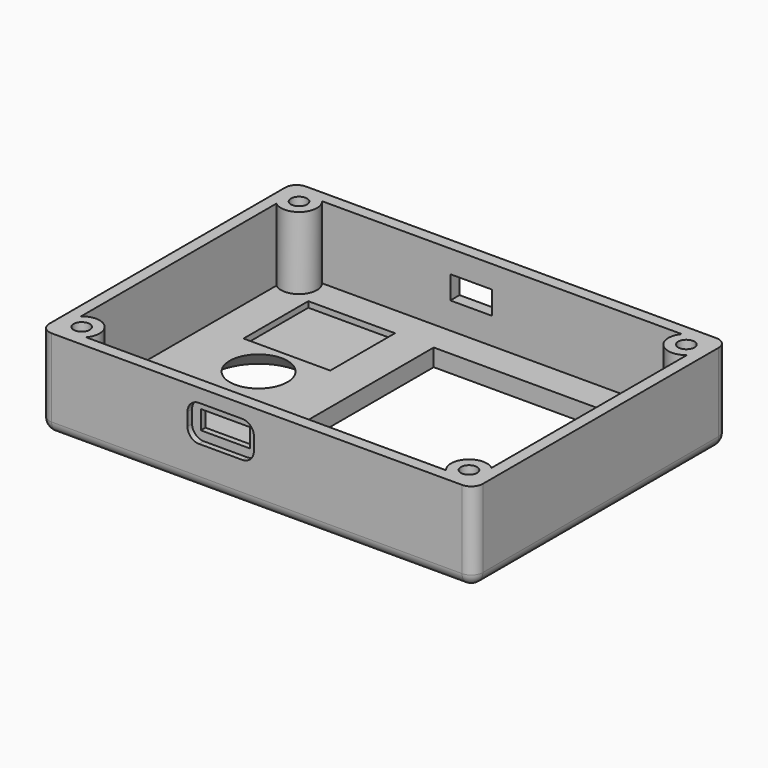
from build123d import *

# Parameters (mm, degrees)
F0_R      = 5
F0_W      = 15
F0_H      = 14
F1_DEPTH  = 3
F0_W_2    = 5
F0_H_2    = 23
F2_DEPTH  = 1
F0_R_2    = 1.4
F3_DEPTH  = 15.5
F4_DEPTH  = 3
F5_R      = 2
F6_W      = 7.25
F6_H      = 4
F7_DEPTH  = 25
F8_W      = 8.5
F8_H      = 3.25
F9_DEPTH  = 25
F8_W_2    = 11.5
F8_H_2    = 6.25
F10_DEPTH = 1
F11_R     = 2
F12_DEPTH = 2
F13_SIZE  = 2.99999


# Not quite as in the source:
# - a fillet or chamfer is up to 0.001 mm smaller than in the source, because OpenCascade refuses the exact size
# - a feature names something its author has since deleted; it is built from what else it names


with BuildPart() as f1:
    # F0 (on Top) → F1 (new body)
    with BuildSketch(Plane.XY):
        with BuildLine():
            ThreePointArc((35.5, 21.1314561435), (31.3079689783, 21.3079689783), (31.1314561435, 25.5))
            Line((31.1314561435, 25.5), (-31.1314561435, 25.5))
            ThreePointArc((-31.1314561435, 25.5), (-31.3079689783, 21.3079689783), (-35.5, 21.1314561435))
            Line((-35.5, 21.1314561435), (-35.5, -21.1314561435))
            ThreePointArc((-35.5, -21.1314561435), (-31.3079689783, -21.3079689783), (-31.1314561435, -25.5))
            Line((-31.1314561435, -25.5), (31.1314561435, -25.5))
            ThreePointArc((31.1314561435, -25.5), (31.3079689783, -21.3079689783), (35.5, -21.1314561435))
            Line((35.5, -21.1314561435), (35.5, 21.1314561435))
        make_face()
        with Locations((-21.7, 0)):
            Circle(F0_R, mode=Mode.SUBTRACT)
        with Locations((-21.8, 13.25)):
            Rectangle(F0_W, F0_H, mode=Mode.SUBTRACT)
        Polygon((-7.6, -20.25), (-7.6, 20.25), (27, 20.25), (27, 11.5), (32, 11.5), (32, -11.5), (27, -11.5), (27, -20.25), align=None, mode=Mode.SUBTRACT)
    extrude(amount=F1_DEPTH)

    # F0 (on Top) → F2 (join)
    with BuildSketch(Plane.XY):
        with Locations((29.5, 0)):
            Rectangle(F0_W_2, F0_H_2)
    extrude(amount=F2_DEPTH)

    # F0 (on Top) → F3 (join)
    with BuildSketch(Plane.XY):
        with BuildLine():
            ThreePointArc((37.5, 25.5), (36.9142135624, 26.9142135624), (35.5, 27.5))
            Line((35.5, 27.5), (-35.5, 27.5))
            ThreePointArc((-35.5, 27.5), (-36.9142135624, 26.9142135624), (-37.5, 25.5))
            Line((-37.5, 25.5), (-37.5, -25.5))
            ThreePointArc((-37.5, -25.5), (-36.9142135624, -26.9142135624), (-35.5, -27.5))
            Line((-35.5, -27.5), (35.5, -27.5))
            ThreePointArc((35.5, -27.5), (36.9142135624, -26.9142135624), (37.5, -25.5))
            Line((37.5, -25.5), (37.5, 25.5))
        make_face()
        Polygon((31.1314561435, 25.5), (35.5, 25.5), (35.5, 21.1314561435), (35.5, -21.1314561435), (35.5, -25.5), (31.1314561435, -25.5), (-31.1314561435, -25.5), (-35.5, -25.5), (-35.5, -21.1314561435), (-35.5, 21.1314561435), (-35.5, 25.5), (-31.1314561435, 25.5), align=None, mode=Mode.SUBTRACT)
        with BuildLine():
            ThreePointArc((-35.5, 21.1314561435), (-31.3079689783, 21.3079689783), (-31.1314561435, 25.5))
            Line((-31.1314561435, 25.5), (-35.5, 25.5))
            Line((-35.5, 25.5), (-35.5, 21.1314561435))
        make_face()
        with Locations((-33.5, 23.5)):
            Circle(F0_R_2, mode=Mode.SUBTRACT)
        with BuildLine():
            ThreePointArc((-31.1314561435, -25.5), (-31.3079689783, -21.3079689783), (-35.5, -21.1314561435))
            Line((-35.5, -21.1314561435), (-35.5, -25.5))
            Line((-35.5, -25.5), (-31.1314561435, -25.5))
        make_face()
        with Locations((-33.5, -23.5)):
            Circle(F0_R_2, mode=Mode.SUBTRACT)
        with BuildLine():
            Line((35.5, -25.5), (35.5, -21.1314561435))
            ThreePointArc((35.5, -21.1314561435), (31.3079689783, -21.3079689783), (31.1314561435, -25.5))
            Line((31.1314561435, -25.5), (35.5, -25.5))
        make_face()
        with Locations((33.5, -23.5)):
            Circle(F0_R_2, mode=Mode.SUBTRACT)
        with BuildLine():
            Line((35.5, 21.1314561435), (35.5, 25.5))
            Line((35.5, 25.5), (31.1314561435, 25.5))
            ThreePointArc((31.1314561435, 25.5), (31.3079689783, 21.3079689783), (35.5, 21.1314561435))
        make_face()
        with Locations((33.5, 23.5)):
            Circle(F0_R_2, mode=Mode.SUBTRACT)
    extrude(amount=F3_DEPTH)

    # F0 (on Top) → F4 (join)
    with BuildSketch(Plane.XY):
        with Locations((33.5, -23.5)):
            Circle(F0_R_2)
        with Locations((33.5, 23.5)):
            Circle(F0_R_2)
        with Locations((-33.5, 23.5)):
            Circle(F0_R_2)
        with Locations((-33.5, -23.5)):
            Circle(F0_R_2)
    extrude(amount=F4_DEPTH)

    # F5
    f5_edges = [f1.edges().sort_by_distance(p)[0] for p in [
        (-37.5, 0, 0),
    ]]
    fillet(f5_edges, radius=F5_R)

    # F6 (on face) → F7 (cut)
    with BuildSketch(Plane(origin=(0, 27.5, 0), x_dir=(-1, 0, 0), z_dir=(0, 1, 0))):
        with Locations((5.3, 9.6)):
            Rectangle(F6_W, F6_H)
    extrude(amount=-F7_DEPTH, mode=Mode.SUBTRACT)

    # F8 (on face) → F9 (cut)
    with BuildSketch(Plane.XZ.offset(27.5)):
        with Locations((-6.25, 10.075)):
            Rectangle(F8_W, F8_H)
    extrude(amount=-F9_DEPTH, mode=Mode.SUBTRACT)

    # F8 (on face) → F10 (cut)
    with BuildSketch(Plane.XZ.offset(27.5)):
        with Locations((-6.25, 10.075)):
            Rectangle(F8_W_2, F8_H_2)
        with Locations((-6.25, 10.075)):
            Rectangle(F8_W, F8_H, mode=Mode.SUBTRACT)
    extrude(amount=-F10_DEPTH, mode=Mode.SUBTRACT)

    # F11
    f11_edges = [f1.edges().sort_by_distance(p)[0] for p in [
        (-0.5, -27, 13.2),
        (-0.5, -27, 6.95),
        (-12, -27, 6.95),
        (-12, -27, 13.2),
    ]]
    fillet(f11_edges, radius=F11_R)

    # F0 (on Top) → F12 (join)
    with BuildSketch(Plane.XY):
        with Locations((-21.8, 13.25)):
            Rectangle(F0_W, F0_H)
    extrude(amount=F12_DEPTH)

    # F13 (size 3 in the source; OpenCascade refuses exactly that, so slightly less here)
    f13_edges = [f1.edges().sort_by_distance(p)[0] for p in [
        (-26.7, 0, 0),
    ]]
    chamfer(f13_edges, length=F13_SIZE)


solid = f1.part
